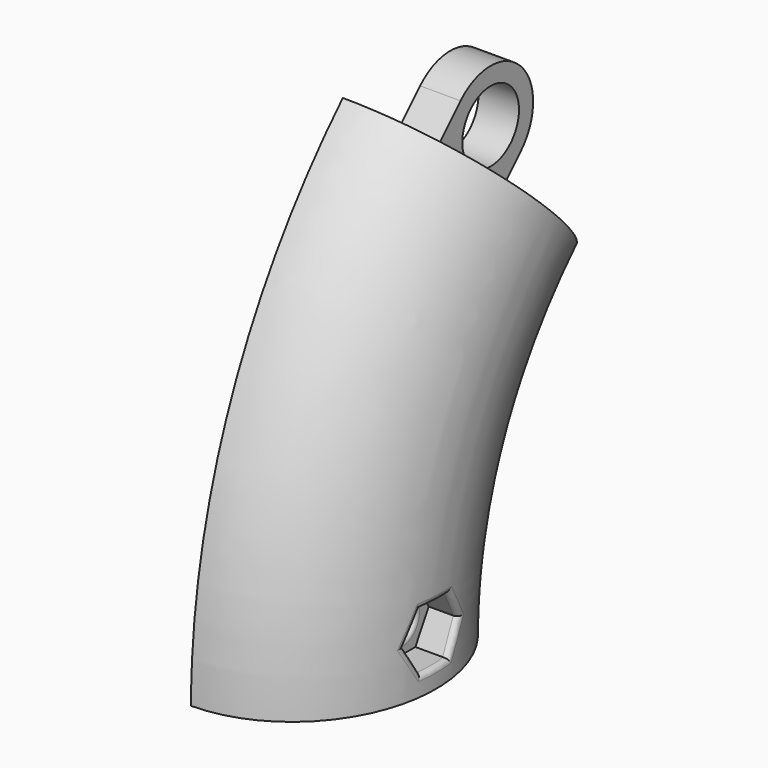
from build123d import *

# Parameters (mm, degrees)
F0_W      = 8.3
F0_H      = 10.8
F1_ANGLE  = 45
F2_W      = 8
F2_H      = 10.5
F3_DEPTH  = 10
F4_R      = 5.24999
F5_R      = 3.5
F6_DEPTH  = 17.0010001
F7_DEPTH  = 10.15
F8_R      = 5.39999
F9_W      = 20
F9_H      = 70
F10_DEPTH = 50
F11_R     = 3.35
F11_R_2   = 1.65
F12_DEPTH = 4.15
F13_DEPTH = 25
F14_R     = 1.65
F15_DEPTH = 25
F16_DEPTH = 5.5
F17_R     = 0.5


# Not quite as in the source:
# - a fillet or chamfer is up to 0.001 mm smaller than in the source, because OpenCascade refuses the exact size


with BuildPart() as f1:
    # F0 (on Top) → F1 (revolve)
    with BuildSketch(Plane.XY):
        with BuildLine():
            add(Edge.make_bspline(
                [(0, 14), (-22.5166604984, 14), (-11.2583302492, -7), (0, -28), (11.2583302492, -7), (22.5166604984, 14), (0, 14)],
                knots=[0, 0, 0, 2.0943951024, 2.0943951024, 4.1887902048, 4.1887902048, 6.2831853072, 6.2831853072, 6.2831853072], degree=2, weights=[1, 0.5, 1, 0.5, 1, 0.5, 1]))
        make_face()
        Rectangle(F0_W, F0_H, mode=Mode.SUBTRACT)
        Rectangle(F0_W, F0_H)
    revolve(axis=Axis((13.7635422871, 50, 0), (-1, 0, 0)), revolution_arc=F1_ANGLE)

    # F2 (on face) → F3 (join)
    with BuildSketch(Plane(origin=(0, 25, 25), x_dir=(1, 0, 0), z_dir=(0, 0.7071067812, 0.7071067812))):
        with Locations((0, -14.6446609407)):
            Rectangle(F2_W, F2_H)
    extrude(amount=F3_DEPTH)

    # F4 (radius 5.25 in the source; OpenCascade refuses exactly that, so slightly less here)
    f4_edges = [f1.edges().sort_by_distance(p)[0] for p in [
        (0, 18.003418, 46.138717),
        (0, 25.428039, 38.714096),
    ]]
    fillet(f4_edges, radius=F4_R)

    # F5 (on face) → F6 (cut, through all)
    with BuildSketch(Plane.YZ.offset(4)):
        with Locations((18.0034181513, 38.71409627)):
            Circle(F5_R)
    extrude(amount=-F6_DEPTH, mode=Mode.SUBTRACT)

    # F0 (on Top) → F7 (cut)
    with BuildSketch(Plane.XY):
        Rectangle(F0_W, F0_H)
    extrude(amount=F7_DEPTH, mode=Mode.SUBTRACT)

    # F8 (radius 5.4 in the source; OpenCascade refuses exactly that, so slightly less here)
    f8_edges = [f1.edges().sort_by_distance(p)[0] for p in [
        (0, 5.4, 10.15),
        (0, -5.4, 10.15),
    ]]
    fillet(f8_edges, radius=F8_R)

    # F9 (on Top) → F10 (intersect)
    with BuildSketch(Plane.XY):
        with Locations((10, 0)):
            Rectangle(F9_W, F9_H)
    extrude(amount=F10_DEPTH, mode=Mode.INTERSECT)

    # F11 (on face) → F12 (join)
    with BuildSketch(Plane(origin=(4.15, 0, 0), x_dir=(0, -1, 0), z_dir=(-1, 0, 0))):
        with Locations((0, 4.75)):
            Circle(F11_R)
        with Locations((0, 4.75)):
            Circle(F11_R_2, mode=Mode.SUBTRACT)
    extrude(amount=F12_DEPTH)

    # F13 (cut): a face of the model
    f13_faces = [f1.faces().sort_by_distance(p)[0] for p in [
        (4.15, 0, 4.75),
    ]]
    extrude(f13_faces, amount=-F13_DEPTH, mode=Mode.SUBTRACT)

    # F14 (on face) → F15 (cut)
    with BuildSketch(Plane(origin=(4.15, 0, 0), x_dir=(0, -1, 0), z_dir=(-1, 0, 0))):
        Polygon((1.6454482672, 7.6), (-1.6454482672, 7.6), (-3.2908965344, 4.75), (-1.6454482672, 1.9), (1.6454482672, 1.9), (3.2908965344, 4.75), align=None)
        with Locations((0, 4.75)):
            Circle(F14_R, mode=Mode.SUBTRACT)
    extrude(amount=-F15_DEPTH, mode=Mode.SUBTRACT)

    # F14 (on face) → F16 (join)
    with BuildSketch(Plane(origin=(4.15, 0, 0), x_dir=(0, -1, 0), z_dir=(-1, 0, 0))):
        Polygon((1.6454482672, 7.6), (-1.6454482672, 7.6), (-3.2908965344, 4.75), (-1.6454482672, 1.9), (1.6454482672, 1.9), (3.2908965344, 4.75), align=None)
        with Locations((0, 4.75)):
            Circle(F14_R, mode=Mode.SUBTRACT)
    extrude(amount=-F16_DEPTH)

    # F17
    f17_edges = [f1.edges().sort_by_distance(p)[0] for p in [
        (12.999956, -0.000217, 1.9),
        (12.77819, -2.469724, 3.327687),
        (12.731462, -2.468902, 6.173737),
        (12.988931, -0.003353, 7.6),
        (12.857066, 2.469489, 6.17272),
        (12.81516, 2.468662, 3.325848),
        (9.65, 1.65, 4.75),
    ]]
    fillet(f17_edges, radius=F17_R)


solid = f1.part
